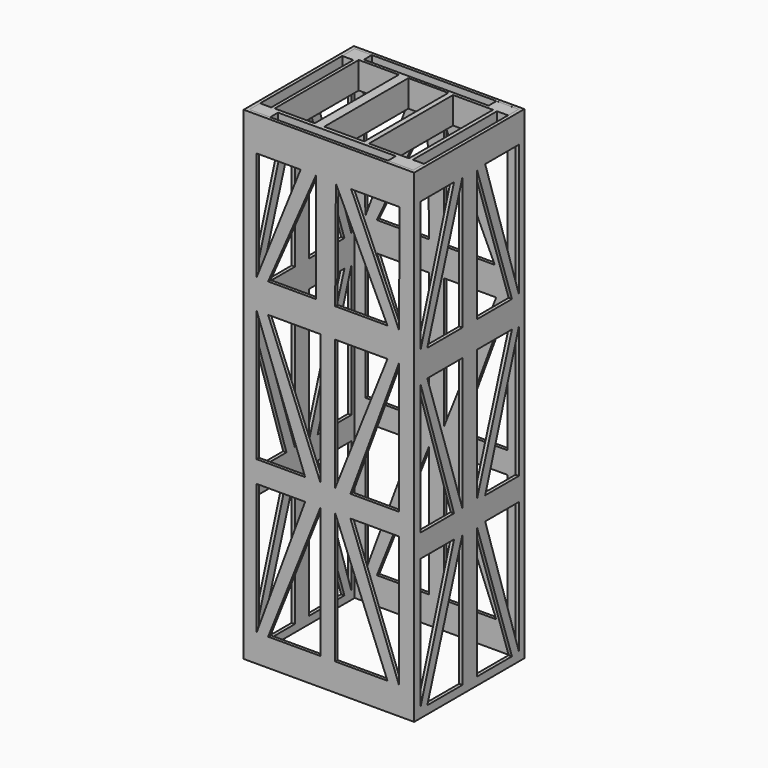
from build123d import *

# Parameters (mm, degrees)
F0_W      = 63.4695142508
F0_H      = 51.2949377298
F0_W_2    = 61
F0_H_2    = 49
F1_DEPTH  = 180
F3_W      = 2.2321660072
F3_H      = 3.732714802
F3_W_2    = 14.8959429935
F3_H_2    = 39.1232501715
F3_W_3    = 3.5938005894
F3_H_3    = 1.2999996543
F3_W_4    = 1.4519924298
F4_DEPTH  = 10
F7_DEPTH  = 5
F10_DEPTH = 5
F13_DEPTH = 5
F16_DEPTH = 5


# Not quite as in the source:
# - ends of sketch curves that miss each other by under 0.0002 mm in the source are joined
# - a feature names something its author has since deleted; it is built from what else it names
# - the program builds the solid bodies; features that only make, move or delete a surface that nothing else refers to are left out


with BuildPart() as f1:
    # F0 (on Top) → F1 (new body)
    with BuildSketch(Plane.XY):
        Rectangle(F0_W, F0_H)
        Rectangle(F0_W_2, F0_H_2, mode=Mode.SUBTRACT)
    extrude(amount=-F1_DEPTH)


with BuildPart() as f4:
    # F3 (on Top) → F4 (new body)
    with BuildSketch(Plane.XY):
        with Locations((-25.2534588799, 22.6865075529)):
            Rectangle(F3_W, F3_H)
        Polygon((-24.1373758763, 20.8201501518), (-26.3695418835, 20.8201501518), (-26.3695418835, 18.7030434608), (-26.3695418835, -19.5201504976), (-22.775741294, -19.5201504976), (-22.775741294, -20.8201501518), (21.0672114044, -20.8201501518), (21.0672114044, -19.5201504976), (10.0216064602, -19.5201504976), (10.0216064602, 19.603099674), (22.2738981247, 19.603099674), (22.2738981247, 20.8201501518), align=None)
        with Locations((-17.7230439149, 0.1456094906)):
            Rectangle(F3_W_2, F3_H_2, mode=Mode.SUBTRACT)
        with Locations((0.6728977896, 0.226427801)):
            Rectangle(F3_W_2, F3_H_2, mode=Mode.SUBTRACT)
        Polygon((-26.3695418835, 18.7030434608), (-26.3695418835, 20.8201501518), (-26.3695418835, 24.5528649539), (-30.5465664715, 24.5528649539), (-30.5465664715, 18.7030434608), align=None)
        Polygon((22.2738981247, 24.4889948517), (22.2738981247, 20.8201501518), (26.3695418835, 20.8201501518), (26.3695418835, 19.603099674), (30.5195916444, 19.603099674), (30.5195916444, 24.4889948517), align=None)
        Polygon((26.3695418835, 20.8201501518), (22.2738981247, 20.8201501518), (22.2738981247, 19.603099674), (24.9175494537, 19.603099674), (26.3695418835, 19.603099674), align=None)
        with Locations((-24.5726415887, -20.1701503247)):
            Rectangle(F3_W_3, F3_H_3)
        Polygon((-26.3695418835, -20.8201501518), (-26.3695418835, -19.5201504976), (-30.8873578906, -19.5201504976), (-30.8873578906, -24.8510874808), (-22.775741294, -24.8510874808), (-22.775741294, -20.8201501518), align=None)
        with Locations((25.6435456686, 0.0414745882)):
            Rectangle(F3_W_4, F3_H_2)
        Polygon((31.1229377985, -19.5201504976), (26.3695418835, -19.5201504976), (26.3695418835, -20.8201501518), (21.0672114044, -20.8201501518), (21.0672114044, -24.8510874808), (31.1229377985, -24.8510874808), align=None)
        Polygon((26.3695418835, -20.8201501518), (26.3695418835, -19.5201504976), (24.9175494537, -19.5201504976), (21.0672114044, -19.5201504976), (21.0672114044, -20.8201501518), align=None)
    extrude(amount=-F4_DEPTH)


with BuildPart() as f7:
    # F6 (on face) → F7 (new body)
    with BuildSketch(Plane.XZ.offset(25.6474688649)):
        Polygon((-4.8192576505, -12.7389919944), (-22.6236060262, -53.3368214965), (-4.8192576505, -53.3368214965), align=None)
    extrude(amount=-F7_DEPTH)


with BuildPart() as f7b:
    # F6 (on face) → F7, piece 2 (new body)
    with BuildSketch(Plane.XZ.offset(25.6474688649)):
        Polygon((-10.5211206246, -12.7389919944), (-26.9000027329, -12.7389919944), (-26.9000027329, -53.3368214965), align=None)
    extrude(amount=-F7_DEPTH)


with BuildPart() as f7c:
    # F6 (on face) → F7, piece 3 (new body)
    with BuildSketch(Plane.XZ.offset(25.6474688649)):
        Polygon((2.3220481817, -53.3368214965), (21.8034163117, -53.3368214965), (2.6015529875, -13.0184972659), align=None)
    extrude(amount=-F7_DEPTH)


with BuildPart() as f7d:
    # F6 (on face) → F7, piece 4 (new body)
    with BuildSketch(Plane.XZ.offset(25.6474688649)):
        Polygon((8.3034159616, -13.0184972659), (26.0798130184, -53.3368214965), (26.3593178242, -13.0184972659), align=None)
    extrude(amount=-F7_DEPTH)


with BuildPart() as f7e:
    # F6 (on face) → F7, piece 5 (new body)
    with BuildSketch(Plane.XZ.offset(25.6474688649)):
        Polygon((-8.8441008702, -112.9688103683), (-26.9000027329, -64.2653927207), (-26.9000027329, -112.9688103683), align=None)
    extrude(amount=-F7_DEPTH)


with BuildPart() as f7f:
    # F6 (on face) → F7, piece 6 (new body)
    with BuildSketch(Plane.XZ.offset(25.6474688649)):
        Polygon((-22.6236060262, -64.2653927207), (-3.1422378961, -112.9688103683), (-3.1422378961, -64.2653927207), align=None)
    extrude(amount=-F7_DEPTH)


with BuildPart() as f7g:
    # F6 (on face) → F7, piece 7 (new body)
    with BuildSketch(Plane.XZ.offset(25.6474688649)):
        Polygon((2.3220481817, -112.9688103683), (21.8034163117, -64.2653927207), (2.3220481817, -64.2653927207), align=None)
    extrude(amount=-F7_DEPTH)


with BuildPart() as f7h:
    # F6 (on face) → F7, piece 8 (new body)
    with BuildSketch(Plane.XZ.offset(25.6474688649)):
        Polygon((26.0798130184, -112.9688103683), (26.0798130184, -64.2653927207), (8.0239111558, -112.9688103683), align=None)
    extrude(amount=-F7_DEPTH)


with BuildPart() as f7i:
    # F6 (on face) → F7, piece 9 (new body)
    with BuildSketch(Plane.XZ.offset(25.6474688649)):
        Polygon((26.0798130184, -169.7498708963), (26.0798130184, -121.0464532487), (8.0239111558, -121.0464532487), align=None)
    extrude(amount=-F7_DEPTH)


with BuildPart() as f7j:
    # F6 (on face) → F7, piece 10 (new body)
    with BuildSketch(Plane.XZ.offset(25.6474688649)):
        Polygon((21.8034163117, -169.7498708963), (2.3220481817, -121.0464532487), (2.3220481817, -169.7498708963), align=None)
    extrude(amount=-F7_DEPTH)


with BuildPart() as f7k:
    # F6 (on face) → F7, piece 11 (new body)
    with BuildSketch(Plane.XZ.offset(25.6474688649)):
        Polygon((-3.1422378961, -169.7498708963), (-3.1422378961, -121.0464532487), (-22.6236060262, -169.7498708963), align=None)
    extrude(amount=-F7_DEPTH)


with BuildPart() as f7l:
    # F6 (on face) → F7, piece 12 (new body)
    with BuildSketch(Plane.XZ.offset(25.6474688649)):
        Polygon((-8.8441008702, -121.0464532487), (-26.9000027329, -121.0464532487), (-26.9000027329, -169.7498708963), align=None)
    extrude(amount=-F7_DEPTH)


with BuildPart() as f1_1:
    add(f1.part)

    # F8: cut F7b, F7, F7c, F7d, F7h, F7g, F7f, F7e, F7l, F7k, F7j, F7i
    add(f7b.part, mode=Mode.SUBTRACT)
    add(f7.part, mode=Mode.SUBTRACT)
    add(f7c.part, mode=Mode.SUBTRACT)
    add(f7d.part, mode=Mode.SUBTRACT)
    add(f7h.part, mode=Mode.SUBTRACT)
    add(f7g.part, mode=Mode.SUBTRACT)
    add(f7f.part, mode=Mode.SUBTRACT)
    add(f7e.part, mode=Mode.SUBTRACT)
    add(f7l.part, mode=Mode.SUBTRACT)
    add(f7k.part, mode=Mode.SUBTRACT)
    add(f7j.part, mode=Mode.SUBTRACT)
    add(f7i.part, mode=Mode.SUBTRACT)


with BuildPart() as f10:
    # F9 (on face) → F10 (new body)
    with BuildSketch(Plane(origin=(-31.7347571254, 0, 0), x_dir=(0, -1, 0), z_dir=(-1, 0, 0))):
        Polygon((-3.3345599659, -60.1282082498), (-3.3345599659, -10.857318528), (-19.7089184076, -60.1282082498), align=None)
    extrude(amount=-F10_DEPTH)


with BuildPart() as f10b:
    # F9 (on face) → F10, piece 2 (new body)
    with BuildSketch(Plane(origin=(-31.7347571254, 0, 0), x_dir=(0, -1, 0), z_dir=(-1, 0, 0))):
        Polygon((19.7089184076, -60.1282082498), (3.3345599659, -10.8271613717), (3.3345599659, -60.1282082498), align=None)
    extrude(amount=-F10_DEPTH)


with BuildPart() as f10c:
    # F9 (on face) → F10, piece 3 (new body)
    with BuildSketch(Plane(origin=(-31.7347571254, 0, 0), x_dir=(0, -1, 0), z_dir=(-1, 0, 0))):
        Polygon((7.2501683608, -10.8271613717), (22.9125972837, -59.7722493112), (22.9125972837, -10.8271613717), align=None)
    extrude(amount=-F10_DEPTH)


with BuildPart() as f10d:
    # F9 (on face) → F10, piece 4 (new body)
    with BuildSketch(Plane(origin=(-31.7347571254, 0, 0), x_dir=(0, -1, 0), z_dir=(-1, 0, 0))):
        Polygon((-3.3345599659, -70.0952149928), (-19.7089184076, -70.0952149928), (-3.3345599659, -119.3962618709), align=None)
    extrude(amount=-F10_DEPTH)


with BuildPart() as f10e:
    # F9 (on face) → F10, piece 5 (new body)
    with BuildSketch(Plane(origin=(-31.7347571254, 0, 0), x_dir=(0, -1, 0), z_dir=(-1, 0, 0))):
        Polygon((-22.9125972837, -70.4511739314), (-22.9125972837, -119.3962618709), (-7.2501683608, -119.3962618709), align=None)
    extrude(amount=-F10_DEPTH)


with BuildPart() as f10f:
    # F9 (on face) → F10, piece 6 (new body)
    with BuildSketch(Plane(origin=(-31.7347571254, 0, 0), x_dir=(0, -1, 0), z_dir=(-1, 0, 0))):
        Polygon((7.2501683608, -119.3962618709), (22.9125972837, -119.3962618709), (22.9125972837, -70.4511739314), align=None)
    extrude(amount=-F10_DEPTH)


with BuildPart() as f10g:
    # F9 (on face) → F10, piece 7 (new body)
    with BuildSketch(Plane(origin=(-31.7347571254, 0, 0), x_dir=(0, -1, 0), z_dir=(-1, 0, 0))):
        Polygon((-7.2501683608, -127.9394105077), (-22.9125972837, -127.9394105077), (-22.9125972837, -176.8844984472), align=None)
    extrude(amount=-F10_DEPTH)


with BuildPart() as f10h:
    # F9 (on face) → F10, piece 8 (new body)
    with BuildSketch(Plane(origin=(-31.7347571254, 0, 0), x_dir=(0, -1, 0), z_dir=(-1, 0, 0))):
        Polygon((-3.3345599659, -127.9394105077), (-19.7089184076, -177.2404573858), (-3.3345599659, -177.2404573858), align=None)
    extrude(amount=-F10_DEPTH)


with BuildPart() as f10i:
    # F9 (on face) → F10, piece 9 (new body)
    with BuildSketch(Plane(origin=(-31.7347571254, 0, 0), x_dir=(0, -1, 0), z_dir=(-1, 0, 0))):
        Polygon((3.3345599659, -127.9394105077), (3.3345599659, -177.2404573858), (19.7089184076, -177.2404573858), align=None)
    extrude(amount=-F10_DEPTH)


with BuildPart() as f10j:
    # F9 (on face) → F10, piece 10 (new body)
    with BuildSketch(Plane(origin=(-31.7347571254, 0, 0), x_dir=(0, -1, 0), z_dir=(-1, 0, 0))):
        Polygon((22.9125972837, -176.8844984472), (22.9125972837, -127.9394105077), (7.2501683608, -127.9394105077), align=None)
    extrude(amount=-F10_DEPTH)


with BuildPart() as f10k:
    # F9 (on face) → F10, piece 11 (new body)
    with BuildSketch(Plane(origin=(-31.7347571254, 0, 0), x_dir=(0, -1, 0), z_dir=(-1, 0, 0))):
        Polygon((3.3345599659, -70.0952149928), (3.3345599659, -119.3962618709), (19.7089184076, -70.0952149928), align=None)
    extrude(amount=-F10_DEPTH)


with BuildPart() as f10l:
    # F9 (on face) → F10, piece 12 (new body)
    with BuildSketch(Plane(origin=(-31.7347571254, 0, 0), x_dir=(0, -1, 0), z_dir=(-1, 0, 0))):
        Polygon((-7.2598186513, -10.857318528), (-22.9125972837, -10.857318528), (-22.9125972837, -59.7722493112), align=None)
    extrude(amount=-F10_DEPTH)


with BuildPart() as f1_2:
    add(f1_1.part)

    # F11: cut F10, F10b, F10c, F10l, F10e, F10d, F10k, F10f, F10j, F10i, F10h, F10g
    add(f10.part, mode=Mode.SUBTRACT)
    add(f10b.part, mode=Mode.SUBTRACT)
    add(f10c.part, mode=Mode.SUBTRACT)
    add(f10l.part, mode=Mode.SUBTRACT)
    add(f10e.part, mode=Mode.SUBTRACT)
    add(f10d.part, mode=Mode.SUBTRACT)
    add(f10k.part, mode=Mode.SUBTRACT)
    add(f10f.part, mode=Mode.SUBTRACT)
    add(f10j.part, mode=Mode.SUBTRACT)
    add(f10i.part, mode=Mode.SUBTRACT)
    add(f10h.part, mode=Mode.SUBTRACT)
    add(f10g.part, mode=Mode.SUBTRACT)


with BuildPart() as f13:
    # F12 (on face) → F13 (new body)
    with BuildSketch(Plane.YZ.offset(31.7347571254)):
        Polygon((-7.0946914335, -10.6470072642), (-22.747470066, -10.6470072642), (-22.747470066, -59.5619380474), align=None)
    extrude(amount=-F13_DEPTH)


with BuildPart() as f13b:
    # F12 (on face) → F13, piece 2 (new body)
    with BuildSketch(Plane.YZ.offset(31.7347571254)):
        Polygon((-3.1694327481, -59.917896986), (-3.1694327481, -10.6470072642), (-19.5437911898, -59.917896986), align=None)
    extrude(amount=-F13_DEPTH)


with BuildPart() as f13c:
    # F12 (on face) → F13, piece 3 (new body)
    with BuildSketch(Plane.YZ.offset(31.7347571254)):
        Polygon((19.8740456253, -59.917896986), (3.4996871836, -10.6168501079), (3.4996871836, -59.917896986), align=None)
    extrude(amount=-F13_DEPTH)


with BuildPart() as f13d:
    # F12 (on face) → F13, piece 4 (new body)
    with BuildSketch(Plane.YZ.offset(31.7347571254)):
        Polygon((7.4152955785, -10.6168501079), (23.0777245015, -59.5619380474), (23.0777245015, -10.6168501079), align=None)
    extrude(amount=-F13_DEPTH)


with BuildPart() as f13e:
    # F12 (on face) → F13, piece 5 (new body)
    with BuildSketch(Plane.YZ.offset(31.7347571254)):
        Polygon((-22.747470066, -70.2408626676), (-22.747470066, -119.1859506071), (-7.085041143, -119.1859506071), align=None)
    extrude(amount=-F13_DEPTH)


with BuildPart() as f13f:
    # F12 (on face) → F13, piece 6 (new body)
    with BuildSketch(Plane.YZ.offset(31.7347571254)):
        Polygon((-3.1694327481, -69.884903729), (-19.5437911898, -69.884903729), (-3.1694327481, -119.1859506071), align=None)
    extrude(amount=-F13_DEPTH)


with BuildPart() as f13g:
    # F12 (on face) → F13, piece 7 (new body)
    with BuildSketch(Plane.YZ.offset(31.7347571254)):
        Polygon((3.4996871836, -69.884903729), (3.4996871836, -119.1859506071), (19.8740456253, -69.884903729), align=None)
    extrude(amount=-F13_DEPTH)


with BuildPart() as f13h:
    # F12 (on face) → F13, piece 8 (new body)
    with BuildSketch(Plane.YZ.offset(31.7347571254)):
        Polygon((7.4152955785, -119.1859506071), (23.0777245015, -119.1859506071), (23.0777245015, -70.2408626676), align=None)
    extrude(amount=-F13_DEPTH)


with BuildPart() as f13i:
    # F12 (on face) → F13, piece 9 (new body)
    with BuildSketch(Plane.YZ.offset(31.7347571254)):
        Polygon((23.0777245015, -176.6741871834), (23.0777245015, -127.7290992439), (7.4152955785, -127.7290992439), align=None)
    extrude(amount=-F13_DEPTH)


with BuildPart() as f13j:
    # F12 (on face) → F13, piece 10 (new body)
    with BuildSketch(Plane.YZ.offset(31.7347571254)):
        Polygon((3.4996871836, -127.7290992439), (3.4996871836, -177.030146122), (19.8740456253, -177.030146122), align=None)
    extrude(amount=-F13_DEPTH)


with BuildPart() as f13k:
    # F12 (on face) → F13, piece 11 (new body)
    with BuildSketch(Plane.YZ.offset(31.7347571254)):
        Polygon((-3.1694327481, -127.7290992439), (-19.5437911898, -177.030146122), (-3.1694327481, -177.030146122), align=None)
    extrude(amount=-F13_DEPTH)


with BuildPart() as f13l:
    # F12 (on face) → F13, piece 12 (new body)
    with BuildSketch(Plane.YZ.offset(31.7347571254)):
        Polygon((-7.085041143, -127.7290992439), (-22.747470066, -127.7290992439), (-22.747470066, -176.6741871834), align=None)
    extrude(amount=-F13_DEPTH)


with BuildPart() as f1_3:
    add(f1_2.part)

    # F14: cut F13, F13b, F13c, F13d, F13e, F13f, F13g, F13h, F13i, F13j, F13k, F13l
    add(f13.part, mode=Mode.SUBTRACT)
    add(f13b.part, mode=Mode.SUBTRACT)
    add(f13c.part, mode=Mode.SUBTRACT)
    add(f13d.part, mode=Mode.SUBTRACT)
    add(f13e.part, mode=Mode.SUBTRACT)
    add(f13f.part, mode=Mode.SUBTRACT)
    add(f13g.part, mode=Mode.SUBTRACT)
    add(f13h.part, mode=Mode.SUBTRACT)
    add(f13i.part, mode=Mode.SUBTRACT)
    add(f13j.part, mode=Mode.SUBTRACT)
    add(f13k.part, mode=Mode.SUBTRACT)
    add(f13l.part, mode=Mode.SUBTRACT)


with BuildPart() as f16:
    # F15 (on face) → F16 (new body)
    with BuildSketch(Plane(origin=(0, 25.6474688649, 0), x_dir=(-1, 0, 0), z_dir=(0, 1, 0))):
        Polygon((-8.6315069348, -13.0680426955), (-26.4470353723, -13.0680426955), (-26.4470353723, -53.8803488016), align=None)
    extrude(amount=-F16_DEPTH)


with BuildPart() as f16b:
    # F15 (on face) → F16, piece 2 (new body)
    with BuildSketch(Plane(origin=(0, 25.6474688649, 0), x_dir=(-1, 0, 0), z_dir=(0, 1, 0))):
        Polygon((-2.6892700698, -13.2785891183), (-21.6376278549, -53.8803488016), (-2.6892700698, -53.8803488016), align=None)
    extrude(amount=-F16_DEPTH)


with BuildPart() as f16c:
    # F15 (on face) → F16, piece 3 (new body)
    with BuildSketch(Plane(origin=(0, 25.6474688649, 0), x_dir=(-1, 0, 0), z_dir=(0, 1, 0))):
        Polygon((2.7750155423, -53.4607544541), (22.2563836724, -53.4607544541), (3.4776383545, -13.0680426955), align=None)
    extrude(amount=-F16_DEPTH)


with BuildPart() as f16d:
    # F15 (on face) → F16, piece 4 (new body)
    with BuildSketch(Plane(origin=(0, 25.6474688649, 0), x_dir=(-1, 0, 0), z_dir=(0, 1, 0))):
        Polygon((11.1019155011, -12.3953102157), (26.5327803791, -53.4607544541), (27.2474437952, -12.3953102157), align=None)
    extrude(amount=-F16_DEPTH)


with BuildPart() as f16e:
    # F15 (on face) → F16, piece 5 (new body)
    with BuildSketch(Plane(origin=(0, 25.6474688649, 0), x_dir=(-1, 0, 0), z_dir=(0, 1, 0))):
        Polygon((-8.3911335096, -113.092743326), (-26.4470353723, -64.3893256783), (-26.4470353723, -113.092743326), align=None)
    extrude(amount=-F16_DEPTH)


with BuildPart() as f16f:
    # F15 (on face) → F16, piece 6 (new body)
    with BuildSketch(Plane(origin=(0, 25.6474688649, 0), x_dir=(-1, 0, 0), z_dir=(0, 1, 0))):
        Polygon((-22.1706386656, -64.3893256783), (-2.6892705355, -113.092743326), (-2.6892705355, -64.3893256783), align=None)
    extrude(amount=-F16_DEPTH)


with BuildPart() as f16g:
    # F15 (on face) → F16, piece 7 (new body)
    with BuildSketch(Plane(origin=(0, 25.6474688649, 0), x_dir=(-1, 0, 0), z_dir=(0, 1, 0))):
        Polygon((2.7750155423, -113.092743326), (22.2563836724, -64.3893256783), (2.7750155423, -64.3893256783), align=None)
    extrude(amount=-F16_DEPTH)


with BuildPart() as f16h:
    # F15 (on face) → F16, piece 8 (new body)
    with BuildSketch(Plane(origin=(0, 25.6474688649, 0), x_dir=(-1, 0, 0), z_dir=(0, 1, 0))):
        Polygon((26.5327803791, -113.092743326), (26.5327803791, -64.3893256783), (8.4768785164, -113.092743326), align=None)
    extrude(amount=-F16_DEPTH)


with BuildPart() as f16i:
    # F15 (on face) → F16, piece 9 (new body)
    with BuildSketch(Plane(origin=(0, 25.6474688649, 0), x_dir=(-1, 0, 0), z_dir=(0, 1, 0))):
        Polygon((26.5327803791, -169.873803854), (26.5327803791, -121.1703862064), (8.4768785164, -121.1703862064), align=None)
    extrude(amount=-F16_DEPTH)


with BuildPart() as f16j:
    # F15 (on face) → F16, piece 10 (new body)
    with BuildSketch(Plane(origin=(0, 25.6474688649, 0), x_dir=(-1, 0, 0), z_dir=(0, 1, 0))):
        Polygon((22.2563836724, -169.873803854), (2.7750155423, -121.1703862064), (2.7750155423, -169.873803854), align=None)
    extrude(amount=-F16_DEPTH)


with BuildPart() as f16k:
    # F15 (on face) → F16, piece 11 (new body)
    with BuildSketch(Plane(origin=(0, 25.6474688649, 0), x_dir=(-1, 0, 0), z_dir=(0, 1, 0))):
        Polygon((-2.6892705355, -169.873803854), (-2.6892705355, -121.1703862064), (-22.1706386656, -169.873803854), align=None)
    extrude(amount=-F16_DEPTH)


with BuildPart() as f16l:
    # F15 (on face) → F16, piece 12 (new body)
    with BuildSketch(Plane(origin=(0, 25.6474688649, 0), x_dir=(-1, 0, 0), z_dir=(0, 1, 0))):
        Polygon((-8.3911335096, -121.1703862064), (-26.4470353723, -121.1703862064), (-26.4470353723, -169.873803854), align=None)
    extrude(amount=-F16_DEPTH)


with BuildPart() as f1_4:
    add(f1_3.part)

    # F17: cut F16d, F16, F16b, F16c, F16e, F16f, F16g, F16h, F16l, F16k, F16j, F16i
    add(f16d.part, mode=Mode.SUBTRACT)
    add(f16.part, mode=Mode.SUBTRACT)
    add(f16b.part, mode=Mode.SUBTRACT)
    add(f16c.part, mode=Mode.SUBTRACT)
    add(f16e.part, mode=Mode.SUBTRACT)
    add(f16f.part, mode=Mode.SUBTRACT)
    add(f16g.part, mode=Mode.SUBTRACT)
    add(f16h.part, mode=Mode.SUBTRACT)
    add(f16l.part, mode=Mode.SUBTRACT)
    add(f16k.part, mode=Mode.SUBTRACT)
    add(f16j.part, mode=Mode.SUBTRACT)
    add(f16i.part, mode=Mode.SUBTRACT)


solid = Compound([f4.part, f1_4.part])
